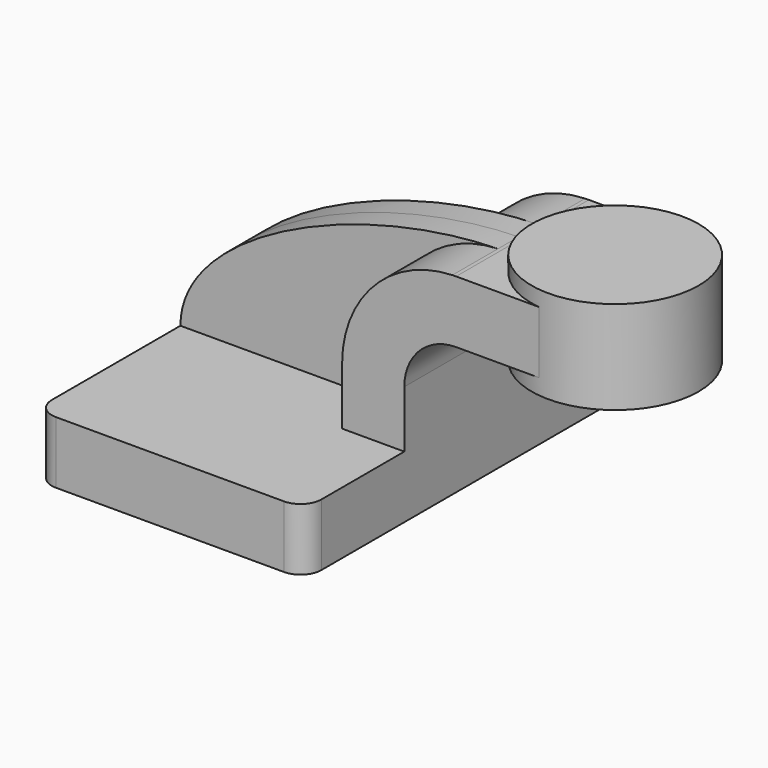
from build123d import *

# Parameters (mm, degrees)
F1_DEPTH = 63.5
F0_W     = 25.2179650775
F0_H     = 19.05
F2_DEPTH = 25.4
F3_DEPTH = 7.9375
F5_R     = 6.35


# Not quite as in the source:
# - a feature names something its author has since deleted; it is built from what else it names


with BuildPart() as f1:
    # F0 (on Front) → F1 (new body, symmetric)
    with BuildSketch(Plane.XZ):
        Polygon((22.225, 9.525), (-41.275, 9.525), (-41.275, -9.525), (41.275, -9.525), (41.275, 9.525), align=None)
    extrude(amount=F1_DEPTH, both=True)

    # F0 (on Front) → F2 (join, symmetric)
    with BuildSketch(Plane.XZ):
        with BuildLine():
            Line((22.225, 27.0002), (22.225, 9.525))
            Line((22.225, 9.525), (41.275, 9.525))
            Line((41.275, 9.525), (41.275, 27.0002))
            ThreePointArc((41.275, 27.0002), (45.9246798487, 38.2255201513), (57.15, 42.8752))
            Line((57.15, 42.8752), (60.325, 42.8752))
            Line((60.325, 42.8752), (60.325, 61.9252))
            Line((60.325, 61.9252), (57.15, 61.9252))
            add(Edge.make_bspline(
                [(56.0083765395, 61.9065364001), (56.3896340439, 61.9145223536), (56.7701888152, 61.920748032), (57.15, 61.9252)],
                knots=[110.545873998, 110.545873998, 110.545873998, 110.545873998, 111.5045361635, 111.5045361635, 111.5045361635, 111.5045361635], degree=3))
            ThreePointArc((56.0083765395, 61.9065364001), (32.0539163976, 51.2889260436), (22.225, 27.0002))
        make_face()
        with Locations((72.9339825387, 52.4002)):
            Rectangle(F0_W, F0_H)
    extrude(amount=F2_DEPTH, both=True)

    # F0 (on Front) → F3 (join, symmetric)
    with BuildSketch(Plane.XZ):
        with BuildLine():
            add(Edge.make_bspline(
                [(-41.275, 9.525), (-41.2634975333, 36.6583816825), (12.04456367, 60.9856549384), (56.0083765395, 61.9065364001)],
                knots=[0, 0, 0, 0, 110.545873998, 110.545873998, 110.545873998, 110.545873998], degree=3))
            Line((-41.275, 9.525), (22.225, 9.525))
            Line((22.225, 9.525), (22.225, 27.0002))
            ThreePointArc((22.225, 27.0002), (32.0539163976, 51.2889260436), (56.0083765395, 61.9065364001))
        make_face()
    extrude(amount=F3_DEPTH, both=True)

    # F0 (on Front) → F4 (revolve)
    with BuildSketch(Plane.XZ):
        Polygon((85.5429650775, 66.675), (85.5429650775, 61.9252), (85.5429650775, 42.8752), (85.5429650775, 38.1), (111.125, 38.1), (111.125, 66.675), align=None)
    revolve(axis=Axis((85.5429650775, 0, 52.3875), (0, 0, -1)))

    # F5
    f5_edges = [f1.edges().sort_by_distance(p)[0] for p in [
        (41.275, -63.5, 0),
        (-41.275, -63.5, 0),
        (41.275, 63.5, 0),
        (-41.275, 63.5, 0),
    ]]
    fillet(f5_edges, radius=F5_R)


solid = f1.part
